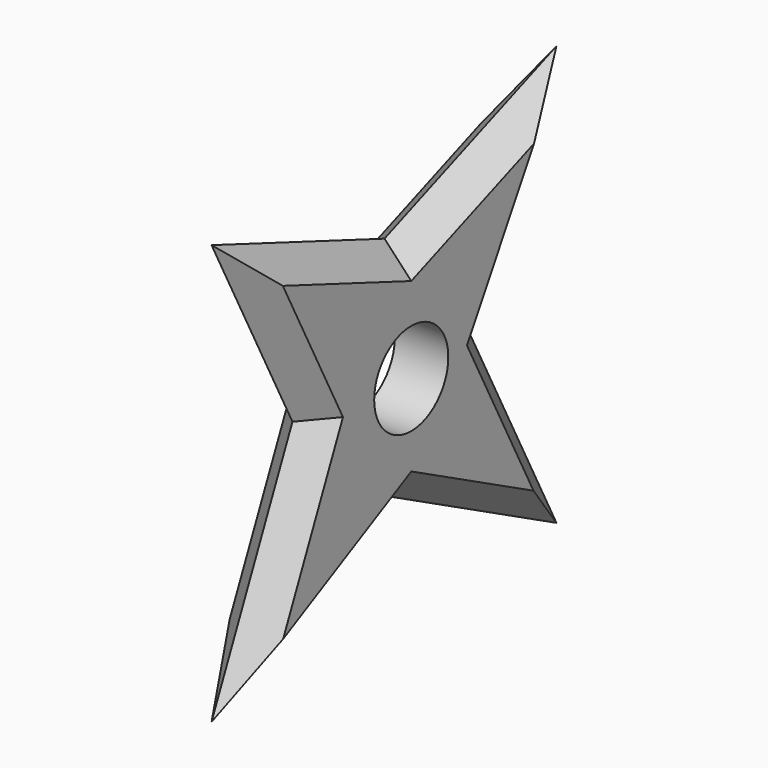
from build123d import *

# Parameters (mm, degrees)
F1_DEPTH = 12.7
F2_SIZE  = 6.34999
F4_D     = 22


# Not quite as in the source:
# - a fillet or chamfer is up to 0.001 mm smaller than in the source, because OpenCascade refuses the exact size


with BuildPart() as f1:
    # F0 (on Right) → F1 (new body)
    with BuildSketch(Plane.YZ):
        Polygon((0, 27.1703749895), (-51.3384975493, 46.6850064695), (-27.3204874247, 0), (0, 0), align=None)
        Polygon((0, 0), (-27.3204874247, 0), (-51.3384975493, -52.9897361994), (0, -26.5776470263), align=None)
        Polygon((23.7766716471, 0), (0, 0), (0, -26.5776470263), (51.0382726789, -52.9897361994), align=None)
        Polygon((51.0382726789, 46.6850064695), (0, 27.1703749895), (0, 0), (23.7766716471, 0), align=None)
    extrude(amount=F1_DEPTH)

    # F2 (size 6.35 in the source; OpenCascade refuses exactly that, so slightly less here)
    f2_edges = [f1.edges().sort_by_distance(p)[0] for p in [
        (12.7, -39.329492, 23.342503),
        (0, -39.329492, 23.342503),
        (0, -25.669249, 36.927691),
        (12.7, -25.669249, 36.927691),
        (0, -39.329492, -26.494868),
        (0, -25.669249, -39.783692),
        (12.7, -25.669249, -39.783692),
        (12.7, -39.329492, -26.494868),
        (0, 25.519136, -39.783692),
        (12.7, 25.519136, -39.783692),
        (0, 37.407472, -26.494868),
        (12.7, 37.407472, -26.494868),
        (0, 37.407472, 23.342503),
        (12.7, 37.407472, 23.342503),
        (0, 25.519136, 36.927691),
        (12.7, 25.519136, 36.927691),
    ]]
    chamfer(f2_edges, length=F2_SIZE)

    # F4 (through all)
    with Locations(Plane(origin=(0, 0, 0), x_dir=(0, 1, 0), z_dir=(-1, 0, 0))):
        with Locations((0, 0)):
            Hole(F4_D / 2)


solid = f1.part
